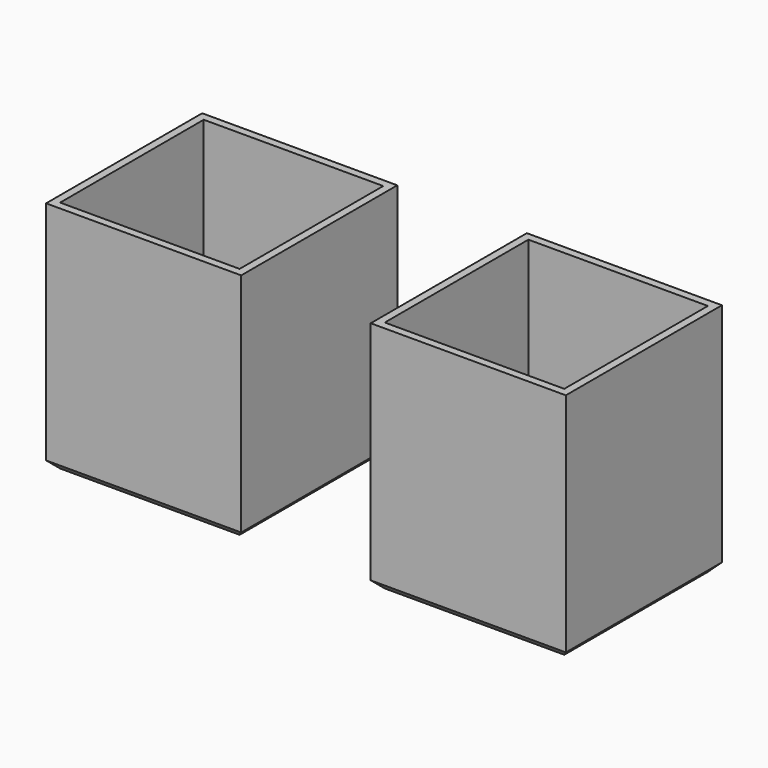
from build123d import *

# Parameters (mm, degrees)
F0_W      = 25
F0_H      = 25
F1_DEPTH  = 30
F2_T      = -1
F4_R      = 1.5
F4_R_2    = 2.5
F5_DEPTH  = 30.001
F7_SIZE   = 1
F7_2_SIZE = 1


# Not quite as in the source:
# - a fillet or chamfer that OpenCascade refuses, or shapes differently, is made with other operations: its cross-section is extruded or revolved along the edge and cut away or added


with BuildPart() as f1:
    # F0 (on Top) → F1 (new body)
    with BuildSketch(Plane.XY):
        Rectangle(F0_W, F0_H)
    extrude(amount=F1_DEPTH)

    # F2
    f2_openings = [f1.faces().sort_by_distance(p)[0] for p in [
        (0, 0, 30),
    ]]
    offset(amount=F2_T, openings=f2_openings)


with BuildPart() as f3_1:
    # F3: copy of F1
    add(f1.part.moved(Location((41.6, 0, 0))))


with BuildPart() as f5_tool:
    # F4 (on face) → F5 (new body, through all)
    with BuildSketch(Plane(origin=(0, 0, 0), x_dir=(1, 0, 0), z_dir=(0, 0, -1))):
        Circle(F4_R)
        with Locations((41.6, 0)):
            Circle(F4_R_2)
    extrude(amount=-F5_DEPTH)


with BuildPart() as f1_1:
    add(f1.part)

    # F5: cut by f5_tool
    add(f5_tool.part, mode=Mode.SUBTRACT)

    # F6: fillet of radius 2 on 1 edges, made by hand

    # F6_s1 → F6_t2 (revolve, cut)
    with BuildSketch(Plane.XZ):
        with BuildLine():
            ThreePointArc((1.5, 0), (2.2320508076, 0.7320508076), (3.2320508076, 1))
            Line((3.2320508076, 1), (1.5, 1))
            Line((1.5, 1), (1.5, 0))
        make_face()
    revolve(axis=Axis((0, 0, 1), (0, 0, -1)), mode=Mode.SUBTRACT)

    # F7
    f7_edges = [f1_1.edges().sort_by_distance(p)[0] for p in [
        (-12.5, 0, 0),
        (0, 12.5, 0),
        (12.5, 0, 0),
        (0, -12.5, 0),
    ]]
    chamfer(f7_edges, length=F7_SIZE)


with BuildPart() as f3_1_1:
    add(f3_1.part)

    # F5: cut by f5_tool
    add(f5_tool.part, mode=Mode.SUBTRACT)

    # F6#2: fillet of radius 2 on 1 edges, made by hand

    # F6_2_s1 → F6_2_t2 (revolve, cut)
    with BuildSketch(Plane.XZ):
        with BuildLine():
            ThreePointArc((44.1, 0), (44.8320508076, 0.7320508076), (45.8320508076, 1))
            Line((45.8320508076, 1), (44.1, 1))
            Line((44.1, 1), (44.1, 0))
        make_face()
    revolve(axis=Axis((41.6, 0, 1), (0, 0, -1)), mode=Mode.SUBTRACT)

    # F7#2
    f7_2_edges = [f3_1_1.edges().sort_by_distance(p)[0] for p in [
        (41.6, -12.5, 0),
        (29.1, 0, 0),
        (54.1, 0, 0),
        (41.6, 12.5, 0),
    ]]
    chamfer(f7_2_edges, length=F7_2_SIZE)


solid = Compound([f1_1.part, f3_1_1.part])
